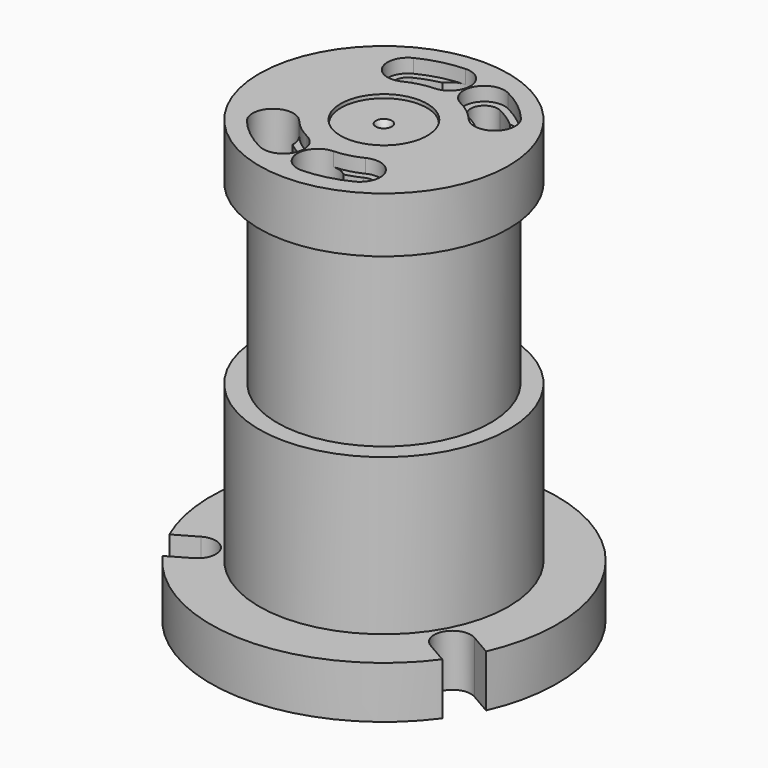
from build123d import *

# Parameters (mm, degrees)
F2_R            = 4.9911
F3_DEPTH        = 20.321
F5_DEPTH        = 20.321
F5_COPIES_COUNT = 2
F7_DEPTH        = 5.08
F7_COPIES_COUNT = 2
F12_D           = 7.9375
F12_DEPTH       = 30.48
F12_CSINK_D     = 9.906
F12_CSINK_ANGLE = 90
F12_TIP         = 2.3846655818
F14_DEPTH       = 25.4


# Not quite as in the source:
# - a pattern or mirror of a feature is missing from the dataset's text; its kind, count and spacing are read off the source's solid


with BuildPart() as f1:
    # F0 (on Front) → F1 (revolve)
    with BuildSketch(Plane.XZ):
        Polygon((-15.875, -14.732), (-15.875, 0), (-45.72, 0), (-45.72, -20.32), (-39.243, -20.32), (-39.243, -14.732), align=None)
    revolve(axis=Axis((0, 0, -19.2851209147), (0, 0, -1)))

    # F2 (on face) → F3 (cut, through all)
    with BuildSketch(Plane.XY):
        with Locations((-13.97, 28.5114292872)):
            Circle(F2_R)
        with Locations((13.97, 28.5114292872)):
            Circle(F2_R)
        with Locations((13.97, -28.5114292872)):
            Circle(F2_R)
        with Locations((-13.97, -28.5114292872)):
            Circle(F2_R)
    extrude(amount=-F3_DEPTH, mode=Mode.SUBTRACT)

    # F4 (on face) → F5 (cut, through all)
    with BuildSketch(Plane.XY):
        with BuildLine():
            ThreePointArc((-11.773916, 24.0294326033), (-8.978607984, 25.2076045645), (-6.0679155964, 26.0618328121))
            ThreePointArc((-6.0679155964, 26.0618328121), (6.2688347989, 32.6637026574), (-7.318549504, 36.0048227654))
            ThreePointArc((-7.318549504, 36.0048227654), (-11.8384597971, 34.7815942539), (-16.166084, 32.9934259712))
            ThreePointArc((-16.166084, 32.9934259712), (-18.451996684, 26.3153452872), (-11.773916, 24.0294326033))
        make_face()
        with BuildLine():
            ThreePointArc((11.773916, 24.0294326033), (14.4179170537, 22.5424576531), (16.876633005, 20.7657888756))
            ThreePointArc((16.876633005, 20.7657888756), (29.6536423348, 15.0624452633), (23.9675734397, 27.847151607))
            ThreePointArc((23.9675734397, 27.847151607), (20.2311307106, 30.6693622265), (16.166084, 32.9934259712))
            ThreePointArc((16.166084, 32.9934259712), (9.488003316, 30.7075132872), (11.773916, 24.0294326033))
        make_face()
    f5 = extrude(amount=-F5_DEPTH, mode=Mode.SUBTRACT)

    # F5_copies: F5 ×2 about axis
    f5_copies_axis = Axis((0, 0, 0), (0, 0, 1))
    for i in range(1, F5_COPIES_COUNT):
        add(f5.rotate(f5_copies_axis, i * 360 / F5_COPIES_COUNT), mode=Mode.SUBTRACT)

    # F6 (on face) → F7 (cut)
    with BuildSketch(Plane.XY):
        with BuildLine():
            ThreePointArc((-6.0679155964, 26.0618328121), (-6.5206277247, 25.952266631), (-6.9713641639, 25.8348371565))
            ThreePointArc((-6.9713641639, 25.8348371565), (-8.4378661433, 23.4576639591), (-10.6730803815, 21.7827317885))
            ThreePointArc((-10.6730803815, 21.7827317885), (-5.9109631603, 23.5257850776), (-0.890508463, 24.240648582))
            ThreePointArc((-0.890508463, 24.240648582), (-3.6519576039, 24.6601458625), (-6.0679155964, 26.0618328121))
        make_face()
        with BuildLine():
            ThreePointArc((-16.166084, 32.9934259712), (-13.4125130079, 34.2054516711), (-10.5690108827, 35.1881292224))
            ThreePointArc((-10.5690108827, 35.1881292224), (-13.9118317745, 36.0042035036), (-17.2669197627, 35.2401267153))
            ThreePointArc((-17.2669197627, 35.2401267153), (-20.6986974634, 25.2145095966), (-10.6730803815, 21.7827317885))
            ThreePointArc((-10.6730803815, 21.7827317885), (-8.4378661433, 23.4576639591), (-6.9713641639, 25.8348371565))
            ThreePointArc((-6.9713641639, 25.8348371565), (-9.4160104878, 25.0475043807), (-11.773916, 24.0294326033))
            ThreePointArc((-11.773916, 24.0294326033), (-18.451996684, 26.3153452872), (-16.166084, 32.9934259712))
        make_face()
        with BuildLine():
            ThreePointArc((-17.2669197627, 35.2401267153), (-13.9118317745, 36.0042035036), (-10.5690108827, 35.1881292224))
            ThreePointArc((-10.5690108827, 35.1881292224), (-8.9530972983, 35.633558312), (-7.318549504, 36.0048227654))
            ThreePointArc((-7.318549504, 36.0048227654), (-4.7584578806, 38.3040312845), (-1.440665747, 39.2165466507))
            ThreePointArc((-1.440665747, 39.2165466507), (-9.562762037, 38.0600398216), (-17.2669197627, 35.2401267153))
        make_face()
        with BuildLine():
            ThreePointArc((30.1075671654, 25.1703684593), (24.2164306207, 30.8800507932), (17.2669198215, 35.2401266865))
            ThreePointArc((17.2669198215, 35.2401266865), (19.9267205597, 33.0570347666), (21.3303084021, 29.9153200331))
            ThreePointArc((21.3303084021, 29.9153200331), (22.6725352574, 28.9113225953), (23.9675734397, 27.847151607))
            ThreePointArc((23.9675734397, 27.847151607), (27.3533197427, 27.2330247473), (30.1075671654, 25.1703684593))
        make_face()
        with BuildLine():
            ThreePointArc((21.3303084021, 29.9153200331), (19.9267205597, 33.0570347666), (17.2669198215, 35.2401266865))
            ThreePointArc((17.2669198215, 35.2401266865), (7.2413025475, 31.808349), (10.673080396, 21.7827317814))
            ThreePointArc((10.673080396, 21.7827317814), (13.3664144509, 21.0427792429), (16.1436191209, 21.3406253632))
            ThreePointArc((16.1436191209, 21.3406253632), (14.023359544, 22.7900003578), (11.773916, 24.0294326033))
            ThreePointArc((11.773916, 24.0294326033), (9.488003316, 30.7075132872), (16.166084, 32.9934259712))
            ThreePointArc((16.166084, 32.9934259712), (18.8112611176, 31.560178776), (21.3303084021, 29.9153200331))
        make_face()
        with BuildLine():
            ThreePointArc((16.1436191209, 21.3406253632), (13.3664144509, 21.0427792429), (10.673080396, 21.7827317814))
            ThreePointArc((10.673080396, 21.7827317814), (14.9687322834, 19.0876688683), (18.6101788379, 15.558383355))
            ThreePointArc((18.6101788379, 15.558383355), (17.2494656652, 17.9976533533), (16.876633005, 20.7657888756))
            ThreePointArc((16.876633005, 20.7657888756), (16.5126276486, 21.0563970648), (16.1436191209, 21.3406253632))
        make_face()
        with BuildLine():
            ThreePointArc((-6.9713641639, 25.8348371565), (-6.6016274755, 27.1504974961), (-6.477, 28.5114292872))
            ThreePointArc((-6.477, 28.5114292872), (-7.5813905873, 32.4268754651), (-10.5690108827, 35.1881292224))
            ThreePointArc((-10.5690108827, 35.1881292224), (-13.4125130079, 34.2054516711), (-16.166084, 32.9934259712))
            ThreePointArc((-16.166084, 32.9934259712), (-18.451996684, 26.3153452872), (-11.773916, 24.0294326033))
            ThreePointArc((-11.773916, 24.0294326033), (-9.4160104878, 25.0475043807), (-6.9713641639, 25.8348371565))
        make_face()
        with BuildLine():
            ThreePointArc((21.463, 28.5114292872), (21.4297533423, 29.216503093), (21.3303084021, 29.9153200331))
            ThreePointArc((21.3303084021, 29.9153200331), (18.8112611176, 31.560178776), (16.166084, 32.9934259712))
            ThreePointArc((16.166084, 32.9934259712), (9.488003316, 30.7075132872), (11.773916, 24.0294326033))
            ThreePointArc((11.773916, 24.0294326033), (14.023359544, 22.7900003578), (16.1436191209, 21.3406253632))
            ThreePointArc((16.1436191209, 21.3406253632), (19.9879721282, 24.047231659), (21.463, 28.5114292872))
        make_face()
    f7 = extrude(amount=-F7_DEPTH, mode=Mode.SUBTRACT)

    # F7_copies: F7 ×2 about axis
    f7_copies_axis = Axis((0, 0, 0), (0, 0, 1))
    for i in range(1, F7_COPIES_COUNT):
        add(f7.rotate(f7_copies_axis, i * 360 / F7_COPIES_COUNT), mode=Mode.SUBTRACT)


with BuildPart() as f9:
    # F8 (on Right) → F9 (revolve)
    with BuildSketch(Plane.YZ):
        Polygon((-39.116, -14.732), (-39.116, -85.09), (-45.72, -85.09), (-45.72, -142.24), (-63.5, -142.24), (-63.5, -161.29), (0, -161.29), (0, -1.27), (-15.748, -1.27), (-15.748, -14.732), align=None)
    revolve(axis=Axis((0, 0, -69.3293474615), (0, 0, -1)))

    # F12
    with Locations(Plane.XY.offset(-14.732)):
        with Locations((-13.97, 28.5114292872), (-13.97, -28.5114292872), (13.97, -28.5114292872), (13.97, 28.5114292872)):
            CounterSinkHole(F12_D / 2, F12_CSINK_D / 2, depth=F12_DEPTH, counter_sink_angle=F12_CSINK_ANGLE)
            with Locations((0, 0, -(F12_DEPTH + F12_TIP / 2))):  # 118° drill point
                Cone(0, F12_D / 2, F12_TIP, mode=Mode.SUBTRACT)

    # F13 (on face) → F14 (cut)
    with BuildSketch(Plane.XY.offset(-142.24)):
        with BuildLine():
            Line((-6.731, 67.5381188877), (-6.731, 53.975))
            ThreePointArc((-6.731, 53.975), (0, 47.244), (6.731, 53.975))
            Line((6.731, 53.975), (6.731, 67.5381188877))
            Line((6.731, 67.5381188877), (-6.731, 67.5381188877))
        make_face()
        with BuildLine():
            Line((67.5437636953, -31.2241208278), (50.1092211693, -21.1582830071))
            ThreePointArc((50.1092211693, -21.1582830071), (40.9145041764, -23.622), (43.3782211693, -32.8167169929))
            Line((43.3782211693, -32.8167169929), (60.8127636953, -42.8825548135))
            Line((60.8127636953, -42.8825548135), (67.5437636953, -31.2241208278))
        make_face()
        with BuildLine():
            Line((-66.4555672965, -46.1404289916), (-43.3782211693, -32.8167169929))
            ThreePointArc((-43.3782211693, -32.8167169929), (-40.9145041764, -23.622), (-50.1092211693, -21.1582830071))
            Line((-50.1092211693, -21.1582830071), (-73.1865672965, -34.4819950059))
            Line((-73.1865672965, -34.4819950059), (-66.4555672965, -46.1404289916))
        make_face()
    extrude(amount=-F14_DEPTH, mode=Mode.SUBTRACT)

    # F15 (on Right) → F16 (revolve, cut)
    with BuildSketch(Plane.YZ):
        Polygon((1.5875, -3.6175851259), (2.9428789044, -1.27), (0, -1.27), (0, -7.3765758425), (1.5875, -6.5038431916), align=None)
    revolve(axis=Axis((0, 0, -4.3232879212), (0, 0, 1)), mode=Mode.SUBTRACT)


solid = Compound([f1.part, f9.part])
